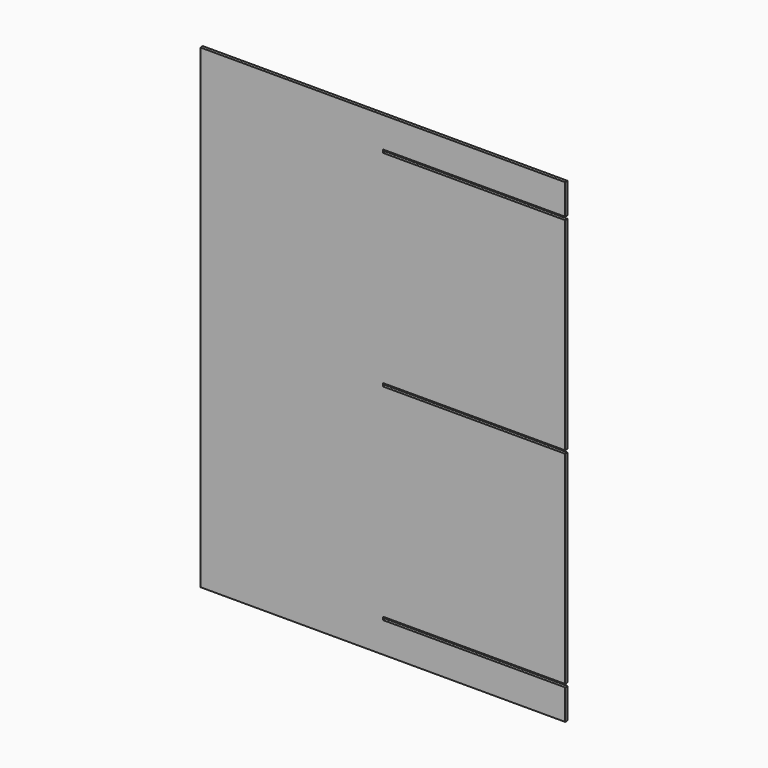
from build123d import *

# Parameters (mm, degrees)
F1_DEPTH = 3


with BuildPart() as f1:
    # F0 (on Front) → F1 (new body)
    with BuildSketch(Plane.XZ):
        Polygon((413.1619042158, 263.3282363415), (233.1619042158, 263.3282363415), (233.1619042158, 266.3282363415), (413.1619042158, 266.3282363415), (413.1619042158, 466.3282363415), (233.1619042158, 466.3282363415), (233.1619042158, 469.3282363415), (413.1619042158, 469.3282363415), (413.1619042158, 669.3282363415), (233.1619042158, 669.3282363415), (233.1619042158, 672.3282363415), (413.1619042158, 672.3282363415), (413.1619042158, 702.3282363415), (53.1619042158, 702.3282363415), (53.1619042158, 233.3282363415), (413.1619042158, 233.3282363415), align=None)
    extrude(amount=F1_DEPTH)


solid = f1.part
